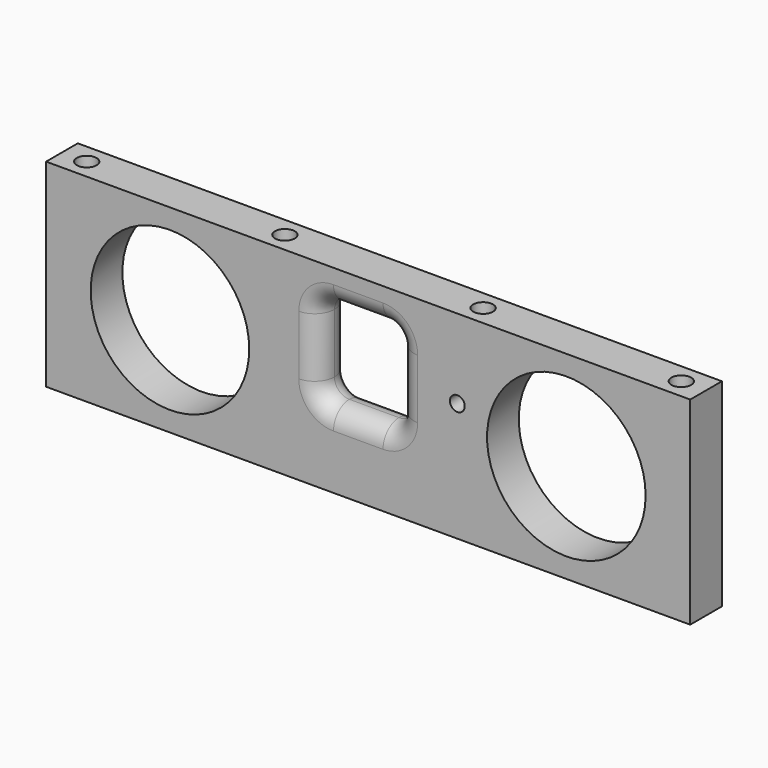
from build123d import *

# Parameters (mm, degrees)
F0_W      = 130
F0_H      = 40
F1_DEPTH  = 8
F2_R      = 16
F3_DEPTH  = 8.001
F4_R      = 2
F5_DEPTH  = 10
F7_DEPTH  = 25
F8_R      = 3.99999
F9_R      = 1.5
F10_DEPTH = 25


# Not quite as in the source:
# - a fillet or chamfer is up to 0.001 mm smaller than in the source, because OpenCascade refuses the exact size


with BuildPart() as f1:
    # F0 (on Front) → F1 (new body)
    with BuildSketch(Plane.XZ):
        Rectangle(F0_W, F0_H)
    extrude(amount=F1_DEPTH)

    # F2 (on face) → F3 (cut, through all)
    with BuildSketch(Plane.XZ.offset(8)):
        with Locations((40, 0)):
            Circle(F2_R)
        with Locations((-40, 0)):
            Circle(F2_R)
    extrude(amount=-F3_DEPTH, mode=Mode.SUBTRACT)

    # F4 (on face) → F5 (cut)
    with BuildSketch(Plane.XY.offset(20)):
        with Locations((-60, -4)):
            Circle(F4_R)
        with Locations((60, -4)):
            Circle(F4_R)
        with Locations((-20, -4)):
            Circle(F4_R)
        with Locations((20, -4)):
            Circle(F4_R)
    extrude(amount=-F5_DEPTH, mode=Mode.SUBTRACT)

    # F6 (on face) → F7 (cut)
    with BuildSketch(Plane.XZ.offset(8)):
        with BuildLine():
            Line((3, 13), (-7, 13))
            ThreePointArc((-7, 13), (-9.1213203436, 12.1213203436), (-10, 10))
            Line((-10, 10), (-10, -2))
            ThreePointArc((-10, -2), (-9.1213203436, -4.1213203436), (-7, -5))
            Line((-7, -5), (3, -5))
            ThreePointArc((3, -5), (5.1213203436, -4.1213203436), (6, -2))
            Line((6, -2), (6, 10))
            ThreePointArc((6, 10), (5.1213203436, 12.1213203436), (3, 13))
        make_face()
    extrude(amount=-F7_DEPTH, mode=Mode.SUBTRACT)

    # F8 (radius 4 in the source; OpenCascade refuses exactly that, so slightly less here)
    f8_edges = [f1.edges().sort_by_distance(p)[0] for p in [
        (6, -8, 4),
        (6, 0, 4),
    ]]
    fillet(f8_edges, radius=F8_R)

    # F9 (on face) → F10 (cut)
    with BuildSketch(Plane(origin=(0, 0, 0), x_dir=(-1, 0, 0), z_dir=(0, 1, 0))):
        with Locations((-18, 4)):
            Circle(F9_R)
    extrude(amount=-F10_DEPTH, mode=Mode.SUBTRACT)


solid = f1.part
